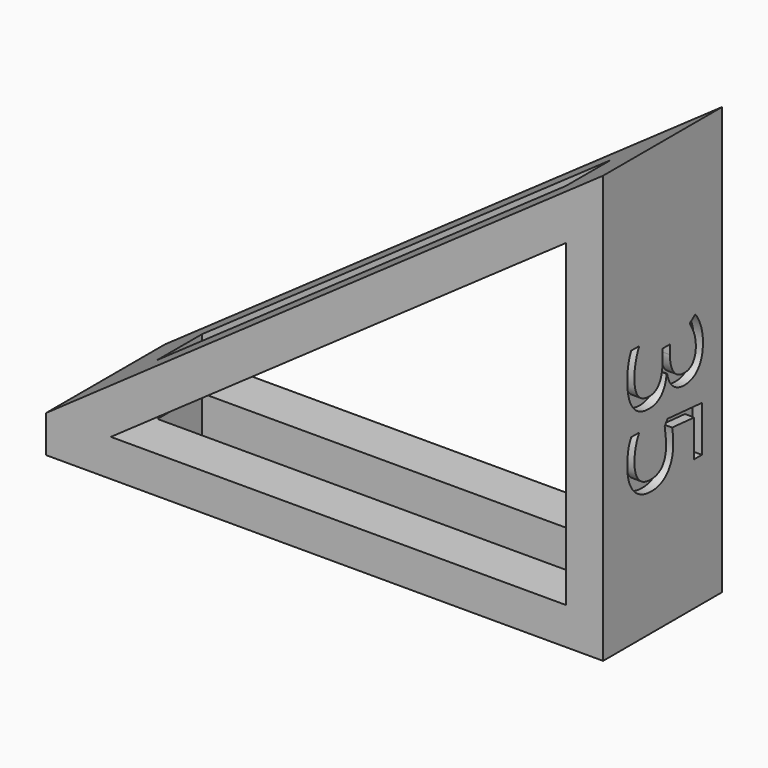
from build123d import *

# Parameters (mm, degrees)
F0_W         = 30
F0_H         = 8
F0_W_2       = 22
F0_H_2       = 3
F1_DEPTH     = 2
F4_DEPTH     = 8
F2_W         = 22
F2_H         = 3
F5_DEPTH     = 25
F7_TEXT_SIZE = 6.9444444444
F8_DEPTH     = 0.5


# Not quite as in the source:
# - Text() gives the source's letters only with a copy of the font that has no kerning and outlines rounded to 1/6400 em; it was checked with that copy


with BuildPart() as f1:
    # F0 (on Top) → F1 (new body)
    with BuildSketch(Plane.XY):
        Rectangle(F0_W, F0_H)
        Rectangle(F0_W_2, F0_H_2, mode=Mode.SUBTRACT)
    extrude(amount=F1_DEPTH)


with BuildPart() as f4:
    # F3 (on face) → F4 (new body)
    with BuildSketch(Plane.XZ.offset(4)):
        Polygon((13, 2), (15, 2), (15, 23.0062261463), (-15, 2), (-11.5131064088, 2), (13, 19.1642618923), align=None)
    extrude(amount=-F4_DEPTH)

    # F2 (on face) → F5 (cut)
    with BuildSketch(Plane.XY.offset(2)):
        Rectangle(F2_W, F2_H)
    extrude(amount=F5_DEPTH, mode=Mode.SUBTRACT)


with BuildPart() as f1_1:
    add(f1.part)

    # F6: union F4
    add(f4.part)

    # F7 (on face) → F8 (cut)
    with BuildSketch(Plane.YZ.offset(15)):
        with Locations(Location((-2.3042319808, 14.2582184014), (0, 0, -90))):
            Text('35', F7_TEXT_SIZE, font='Open Sans', text_align=(TextAlign.LEFT, TextAlign.BOTTOM))
    extrude(amount=-F8_DEPTH, mode=Mode.SUBTRACT)


solid = f1_1.part
